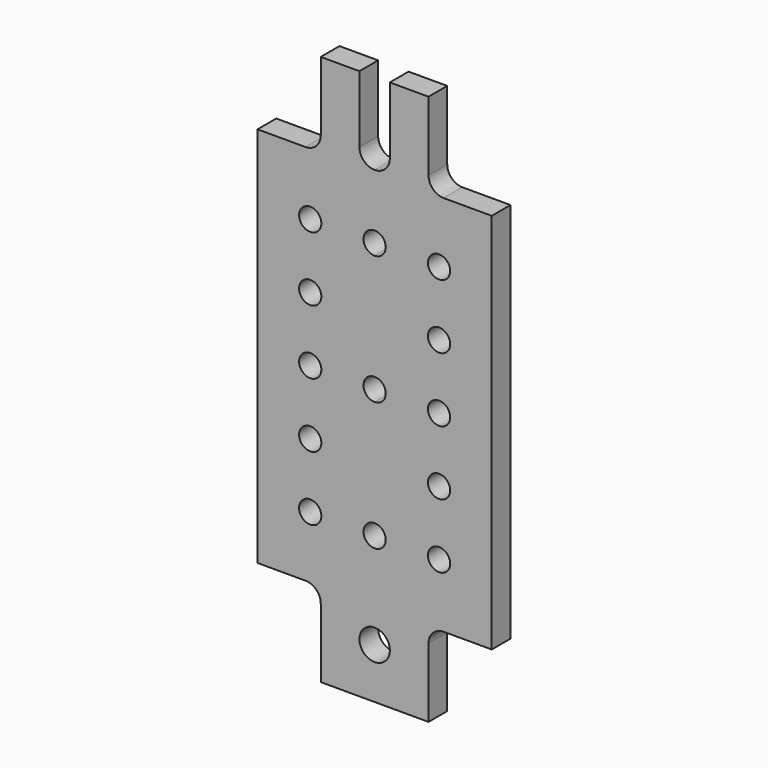
from build123d import *

# Parameters (mm, degrees)
F1_DEPTH = 10
F3_D     = 9.5
F7_D     = 13
F8_R     = 6.49999
F9_R     = 6.5


# Not quite as in the source:
# - a fillet or chamfer is up to 0.001 mm smaller than in the source, because OpenCascade refuses the exact size


with BuildPart() as f1:
    # F0 (on Front) → F1 (new body)
    with BuildSketch(Plane.XZ):
        Polygon((-23, 0), (0, 0), (0, 200), (-6.5, 200), (-6.5, 235), (-23, 235), (-23, 199), (-50, 199), (-50, 36), (-23, 36), align=None)
    extrude(amount=F1_DEPTH)

    # F3 (through all)
    with Locations(Plane.XZ.offset(10)):
        with Locations((-27.5, 172.5), (-27.5, 145), (-27.5, 117.5), (-27.5, 90), (-27.5, 62.5), (0, 62.5), (0, 117.5), (0, 172.5)):
            Hole(F3_D / 2)

    # F4: F1 across face


with BuildPart() as f1_1:
    add(f1.part)
    add(f1.part.mirror(Plane(origin=(0, -5, 90), x_dir=(0, 1, 0), z_dir=(1, 0, 0))))

    # F7 (through all)
    with Locations(Plane.XZ.offset(10)):
        with Locations((0, 21.5)):
            Hole(F7_D / 2)

    # F8 (radius 6.5 in the source; OpenCascade refuses exactly that, so slightly less here)
    f8_edges = [f1_1.edges().sort_by_distance(p)[0] for p in [
        (-6.5, -5, 200),
        (6.5, -5, 200),
    ]]
    fillet(f8_edges, radius=F8_R)

    # F9
    f9_edges = [f1_1.edges().sort_by_distance(p)[0] for p in [
        (23, -5, 199),
        (-23, -5, 199),
        (23, -5, 36),
        (-23, -5, 36),
    ]]
    fillet(f9_edges, radius=F9_R)


solid = f1_1.part
